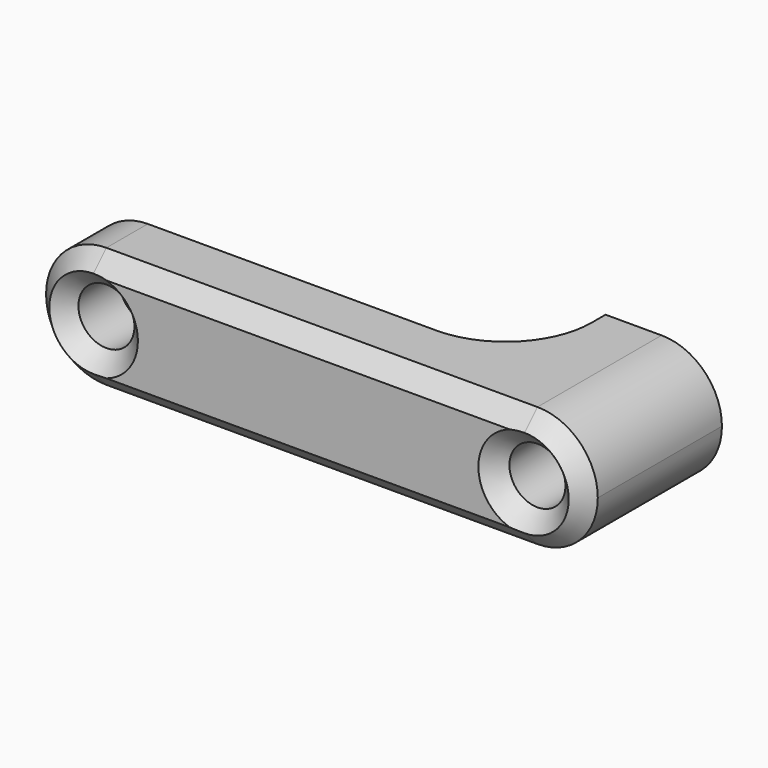
from build123d import *

# Parameters (mm, degrees)
F0_R        = 1.625
F1_DEPTH    = 10
F2_W        = 7.875
F2_H        = 2
F2_H_2      = 4
F2_W_2      = 3.5925165284
F1_FACE1_W  = 25
F1_FACE1_H  = 10
F3_DEPTH    = 25
F4_T1_DEPTH = 25
F4_T4_ANGLE = 180
F4_T6_ANGLE = 180


# Not quite as in the source:
# - a fillet or chamfer that OpenCascade refuses, or shapes differently, is made with other operations: its cross-section is extruded or revolved along the edge and cut away or added


with BuildPart() as f1:
    # F0 (on Front) → F1 (new body)
    with BuildSketch(Plane.XZ):
        with BuildLine():
            ThreePointArc((0, -3.5), (2.4748737342, -2.4748737342), (3.5, 0))
            ThreePointArc((3.5, 0), (2.4748737342, 2.4748737342), (0, 3.5))
            ThreePointArc((0, 3.5), (-3.5, 0), (0, -3.5))
        make_face()
        Circle(F0_R, mode=Mode.SUBTRACT)
        with BuildLine():
            ThreePointArc((0, 3.5), (2.4748737342, 2.4748737342), (3.5, 0))
            Line((3.5, 0), (21.5, 0))
            ThreePointArc((21.5, 0), (22.5251262658, 2.4748737342), (25, 3.5))
            Line((25, 3.5), (0, 3.5))
        make_face()
        with BuildLine():
            Line((21.5, 0), (3.5, 0))
            ThreePointArc((3.5, 0), (2.4748737342, -2.4748737342), (0, -3.5))
            Line((0, -3.5), (25, -3.5))
            ThreePointArc((25, -3.5), (22.5251262658, -2.4748737342), (21.5, 0))
        make_face()
        with BuildLine():
            ThreePointArc((25, 3.5), (22.5251262658, 2.4748737342), (21.5, 0))
            ThreePointArc((21.5, 0), (22.5251262658, -2.4748737342), (25, -3.5))
            ThreePointArc((25, -3.5), (27.4748737342, -2.4748737342), (28.5, 0))
            ThreePointArc((28.5, 0), (27.4748737342, 2.4748737342), (25, 3.5))
        make_face()
        with BuildLine():
            ThreePointArc((26.625, 0), (25, -1.625), (23.375, 0))
            ThreePointArc((23.375, 0), (25, 1.625), (26.625, 0))
        make_face(mode=Mode.SUBTRACT)
    extrude(amount=F1_DEPTH)

    # F2 (on face) + F1_face1 (on face) → F3 (cut)
    with BuildSketch(Plane.XY.offset(3.5)):
        with Locations((3.9375, -5)):
            Rectangle(F2_W, F2_H)
        with Locations((3.9375, -2)):
            Rectangle(F2_W, F2_H_2)
        with Locations((11.8125, -5)):
            Rectangle(F2_W, F2_H)
        with Locations((-1.7962582642, -2)):
            Rectangle(F2_W_2, F2_H_2)
        with Locations((-1.7962582642, -5)):
            Rectangle(F2_W_2, F2_H)
        with Locations((11.8125, -2)):
            Rectangle(F2_W, F2_H_2)
        with BuildLine():
            Line((21.75, 0), (15.75, 0))
            Line((15.75, 0), (15.75, -4))
            Line((15.75, -4), (20.75, -4))
            ThreePointArc((20.75, -4), (21.4934164903, -2.5811388301), (21.75, -1))
            Line((21.75, -1), (21.75, 0))
        make_face()
        with BuildLine():
            Line((20.75, -4), (15.75, -4))
            Line((15.75, -4), (15.75, -6))
            Line((15.75, -6), (16.75, -6))
            ThreePointArc((16.75, -6), (18.9860679775, -5.472135955), (20.75, -4))
        make_face()
    with BuildSketch(Plane(origin=(12.5, -5, -3.5), x_dir=(1, 0, 0), z_dir=(0, 0, -1))):
        Rectangle(F1_FACE1_W, F1_FACE1_H)
    extrude(amount=-F3_DEPTH, dir=(0, 0, 1), mode=Mode.SUBTRACT)

    # F4: chamfer of 1 on 6 edges, made by hand

    # F4_s2 → F4_t1 (cut)
    with BuildSketch(Plane.YZ):
        Polygon((-9, 3.5), (-10, 2.5), (-10, 3.5), align=None)
        Polygon((-10, -2.5), (-9, -3.5), (-10, -3.5), align=None)
    extrude(amount=F4_T1_DEPTH, mode=Mode.SUBTRACT)

    # F4_s3 → F4_t4 (revolve, cut)
    with BuildSketch(Plane.YZ):
        Polygon((-9, 3.5), (-10, 2.5), (-10, 3.5), align=None)
    revolve(axis=Axis((0, -10, 0), (0, -1, 0)), revolution_arc=F4_T4_ANGLE, mode=Mode.SUBTRACT)

    # F4_s5 → F4_t6 (revolve, cut)
    with BuildSketch(Plane.YZ.offset(25)):
        Polygon((-10, -2.5), (-9, -3.5), (-10, -3.5), align=None)
    revolve(axis=Axis((25, -10, 0), (0, -1, 0)), revolution_arc=F4_T6_ANGLE, mode=Mode.SUBTRACT)

    # F4_s7 → F4_t8 (revolve, cut)
    with BuildSketch(Plane.XY):
        Polygon((2.625, -10), (1.625, -9), (1.625, -10), align=None)
    revolve(axis=Axis((0, -10, 0), (0, -1, 0)), mode=Mode.SUBTRACT)

    # F4_s9 → F4_t10 (revolve, cut)
    with BuildSketch(Plane.XY):
        Polygon((22.375, -10), (23.375, -9), (23.375, -10), align=None)
    revolve(axis=Axis((25, -10, 0), (0, 1, 0)), mode=Mode.SUBTRACT)


solid = f1.part
